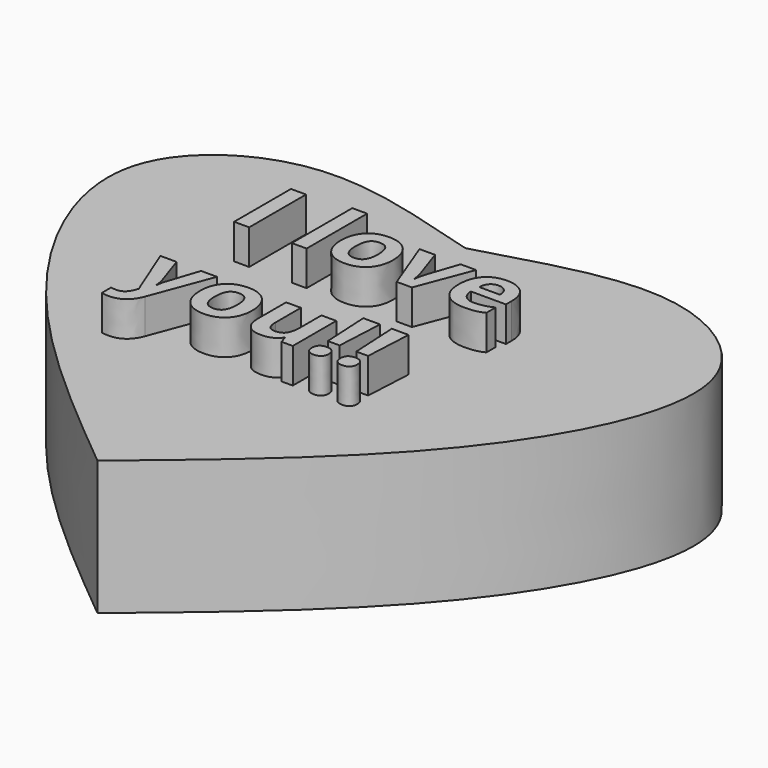
from build123d import *

# Parameters (mm, degrees)
F1_DEPTH     = 25.4
F2_TEXT_SIZE = 18.8366164542
F3_DEPTH     = 6.604


# Not quite as in the source:
# - Text() gives the source's letters only with a copy of the font that has no kerning and outlines rounded to 1/6400 em; it was checked with that copy


with BuildPart() as f1:
    # F0 (on Top) → F1 (new body)
    with BuildSketch(Plane.XY):
        with BuildLine():
            add(Edge.make_bspline(
                [(0, 52.3335896432), (11.7382564908, 55.5838697256), (33.4377219186, 63.368582907), (62.5687317674, 44.0212342242), (44.1873850359, 1.8487209942), (15.7875606387, -21.6777862916), (0, -34.7213223577)],
                knots=[0, 0, 0, 0, 0.2373813559, 0.4409143682, 0.688896759, 1, 1, 1, 1], degree=3))
            add(Edge.make_bspline(
                [(0, 52.3335896432), (-11.7382564908, 55.5838697256), (-33.4377219186, 63.368582907), (-62.5687317674, 44.0212342242), (-44.1873850359, 1.8487209942), (-15.7875606387, -21.6777862916), (0, -34.7213223577)],
                knots=[0, 0, 0, 0, 0.2373813559, 0.4409143682, 0.688896759, 1, 1, 1, 1], degree=3))
        make_face()
    extrude(amount=F1_DEPTH)

    # F2 (on face) → F3 (join)
    with BuildSketch(Plane.XY.offset(25.4)):
        with Locations((-25.7375204044, 27.6750790096)):
            Text('I love', F2_TEXT_SIZE, font='Open Sans', font_style=FontStyle.BOLD, text_align=(TextAlign.LEFT, TextAlign.BOTTOM))
        with Locations((-25.7375204044, 2.0572806319)):
            Text('you!!', F2_TEXT_SIZE, font='Open Sans', font_style=FontStyle.BOLD, text_align=(TextAlign.LEFT, TextAlign.BOTTOM))
    extrude(amount=F3_DEPTH)


solid = f1.part
